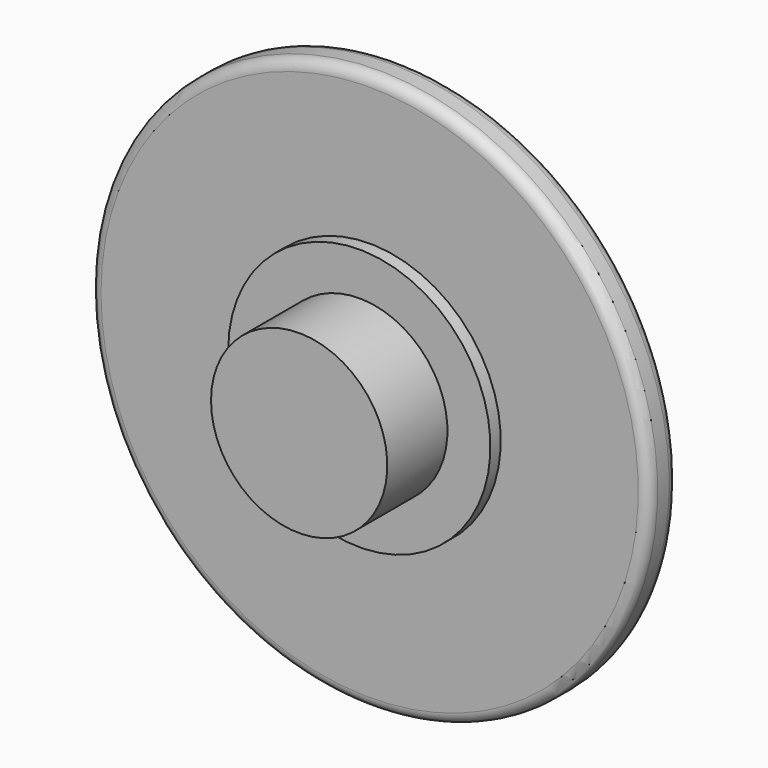
from build123d import *

# Parameters (mm, degrees)
F2_R = 0.5


with BuildPart() as f1:
    # F0 (on Top) → F1 (revolve)
    with BuildSketch(Plane.XY):
        with BuildLine():
            ThreePointArc((0, 14.924920715), (-6.5431261642, 15.3011606257), (-13, 16.424920715))
            Line((-13, 16.424920715), (-13, 14.624920715))
            Line((-13, 14.624920715), (-6.1, 14.624920715))
            Line((-6.1, 14.624920715), (-6.1, 14.024920715))
            Line((-6.1, 14.024920715), (-4.1, 14.024920715))
            Line((-4.1, 14.024920715), (-4.1, 10.524920715))
            Line((-4.1, 10.524920715), (0, 10.524920715))
            Line((0, 10.524920715), (0, 14.924920715))
        make_face()
    revolve(axis=Axis((0, 12.724920715, 0), (0, 1, 0)))

    # F2
    f2_edges = [f1.edges().sort_by_distance(p)[0] for p in [
        (13, 14.624921, 0),
        (13, 16.424921, 0),
    ]]
    fillet(f2_edges, radius=F2_R)


solid = f1.part
